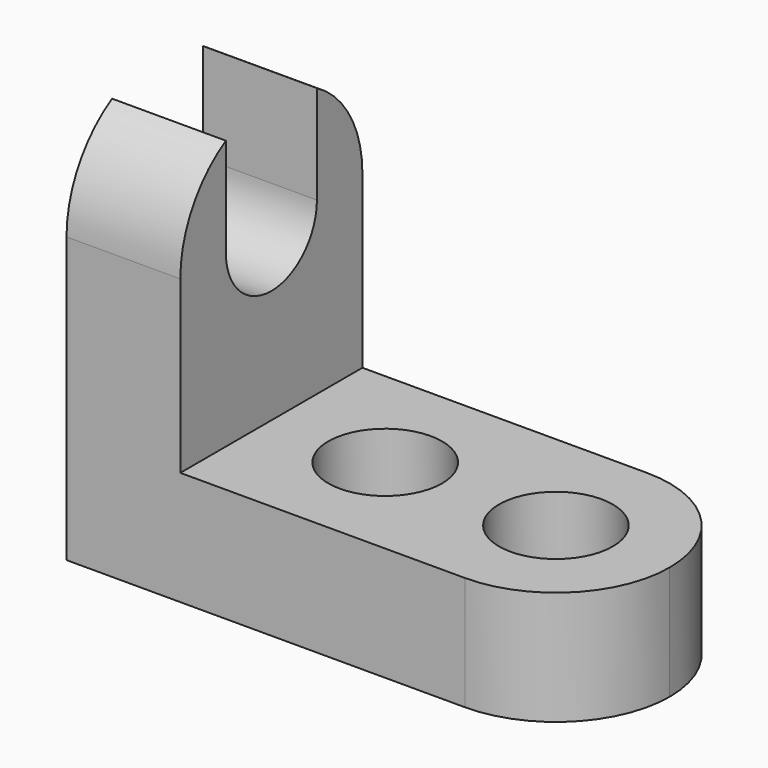
from build123d import *

# Parameters (mm, degrees)
F0_W     = 57.15
F0_H     = 44.45
F1_DEPTH = 25.4
F2_W     = 44.45
F2_H     = 31.75
F3_DEPTH = 25.4
F4_R     = 6.35
F5_DEPTH = 12.7
F7_DEPTH = 12.7


# Not quite as in the source:
# - ends of sketch curves that miss each other by under 0.0002 mm in the source are joined


with BuildPart() as f1:
    # F0 (on Front) → F1 (new body)
    with BuildSketch(Plane.XZ):
        with Locations((28.575, 22.225)):
            Rectangle(F0_W, F0_H)
    extrude(amount=F1_DEPTH)

    # F2 (on face) → F3 (cut)
    with BuildSketch(Plane.XZ.offset(25.4)):
        with Locations((34.925, 28.575)):
            Rectangle(F2_W, F2_H)
    extrude(amount=-F3_DEPTH, mode=Mode.SUBTRACT)

    # F4 (on face) → F5 (cut)
    with BuildSketch(Plane.XY.offset(12.7)):
        with BuildLine():
            ThreePointArc((57.1500001164, -12.7), (53.4302561963, -21.6802561622), (44.45, -25.4))
            Line((44.45, -25.4), (57.15, -25.4))
            Line((57.15, -25.4), (57.1500001164, -12.7))
        make_face()
        with Locations((44.45, -12.7)):
            Circle(F4_R)
        with Locations((25.4, -12.7)):
            Circle(F4_R)
        with BuildLine():
            ThreePointArc((44.45, 0), (53.4302561963, -3.7197438378), (57.1500001164, -12.7))
            Line((57.1500001164, -12.7), (57.15, 0))
            Line((57.15, 0), (44.45, 0))
        make_face()
    extrude(amount=-F5_DEPTH, mode=Mode.SUBTRACT)

    # F6 (on face) → F7 (cut)
    with BuildSketch(Plane.YZ.offset(12.7)):
        with BuildLine():
            Line((-12.7, 44.45), (-19.05, 44.45))
            Line((-19.05, 44.45), (-19.05, 42.7485226281))
            ThreePointArc((-19.05, 42.7485226281), (-15.9870018728, 44.0172579939), (-12.7, 44.45))
        make_face()
        with BuildLine():
            ThreePointArc((-12.7, 44.45), (-15.9870018728, 44.0172579939), (-19.05, 42.7485226281))
            Line((-19.05, 42.7485226281), (-19.05, 31.75))
            Line((-19.05, 31.75), (-6.35, 31.75))
            Line((-6.35, 31.75), (-6.35, 42.7485226281))
            ThreePointArc((-6.35, 42.7485226281), (-9.4129981272, 44.0172579939), (-12.7, 44.45))
        make_face()
        with BuildLine():
            Line((-6.35, 31.75), (-19.05, 31.75))
            ThreePointArc((-19.05, 31.75), (-12.7, 25.4), (-6.35, 31.75))
        make_face()
        with BuildLine():
            Line((-6.35, 44.45), (-6.35, 42.7485226281))
            ThreePointArc((-6.35, 42.7485226281), (-1.7014773719, 38.1), (0, 31.75))
            Line((0, 31.75), (0, 44.45))
            Line((0, 44.45), (-6.35, 44.45))
        make_face()
        with BuildLine():
            Line((-19.05, 44.45), (-25.4, 44.45))
            Line((-25.4, 44.45), (-25.4, 31.75))
            ThreePointArc((-25.4, 31.75), (-23.6985226281, 38.1), (-19.05, 42.7485226281))
            Line((-19.05, 42.7485226281), (-19.05, 44.45))
        make_face()
        with BuildLine():
            Line((-6.35, 44.45), (-12.7, 44.45))
            ThreePointArc((-12.7, 44.45), (-9.4129981272, 44.0172579939), (-6.35, 42.7485226281))
            Line((-6.35, 42.7485226281), (-6.35, 44.45))
        make_face()
    extrude(amount=-F7_DEPTH, mode=Mode.SUBTRACT)


solid = f1.part
